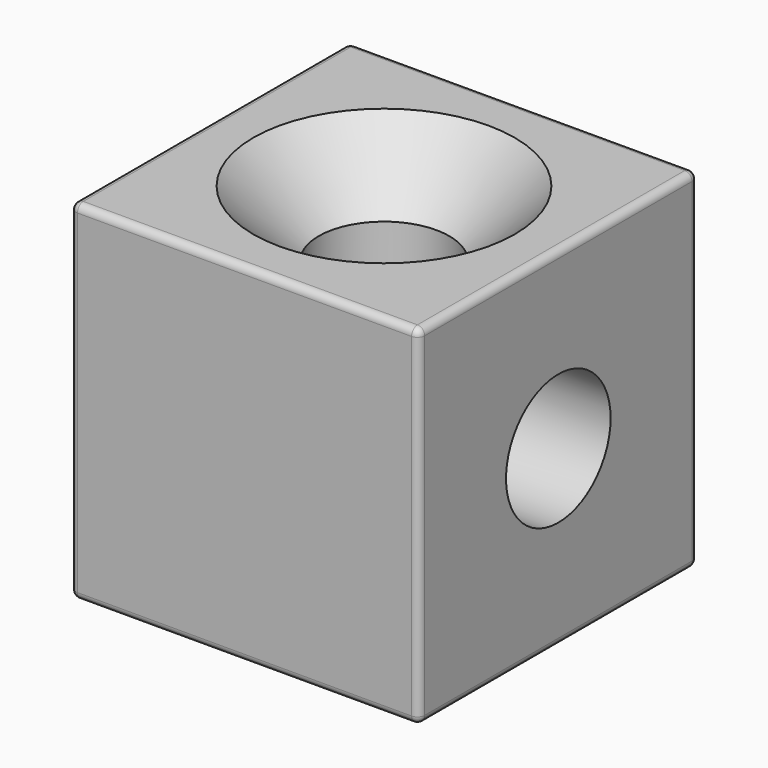
from build123d import *

# Parameters (mm, degrees)
F0_W           = 48
F0_H           = 48
F1_DEPTH       = 48
F2_R           = 1
F3_R           = 1
F4_T1_DEPTH    = 46
F4_T3_DEPTH    = 46
F4_T5_DEPTH    = 46
F4_S9_W        = 1
F4_S9_H        = 1
F4_T10_DEPTH   = 1
F4_S15_W       = 1
F4_S15_H       = 1
F4_T16_DEPTH   = 1
F4_S21_W       = 1
F4_S21_H       = 1
F4_T22_DEPTH   = 1
F4_S27_W       = 1
F4_S27_H       = 1
F4_T28_DEPTH   = 1
F4_T32_ANGLE   = 90
F4_T34_ANGLE   = 90
F6_D           = 18
F6_CSINK_D     = 36
F6_CSINK_ANGLE = 90
F8_D           = 18
F8_CSINK_D     = 36
F8_CSINK_ANGLE = 90


# Not quite as in the source:
# - a fillet or chamfer that OpenCascade refuses, or shapes differently, is made with other operations: its cross-section is extruded or revolved along the edge and cut away or added


with BuildPart() as f1:
    # F0 (on Front) → F1 (new body)
    with BuildSketch(Plane.XZ):
        Rectangle(F0_W, F0_H)
    extrude(amount=F1_DEPTH)

    # F2
    f2_edges = [f1.edges().sort_by_distance(p)[0] for p in [
        (24, -24, 24),
    ]]
    fillet(f2_edges, radius=F2_R)

    # F3
    f3_edges = [f1.edges().sort_by_distance(p)[0] for p in [
        (-24, -24, 24),
        (-0.5, 0, 24),
        (-0.5, -48, 24),
    ]]
    fillet(f3_edges, radius=F3_R)

    # F4: fillet of radius 1 on 8 edges, made by hand

    # F4_s2 → F4_t1 (cut)
    with BuildSketch(Plane.XY.offset(-23)):
        with BuildLine():
            ThreePointArc((-23, -48), (-23.7071067812, -47.7071067812), (-24, -47))
            Line((-24, -47), (-24, -48))
            Line((-24, -48), (-23, -48))
        make_face()
        with BuildLine():
            ThreePointArc((-23, 0), (-23.7071067812, -0.2928932188), (-24, -1))
            Line((-24, -1), (-24, 0))
            Line((-24, 0), (-23, 0))
        make_face()
    extrude(amount=F4_T1_DEPTH, mode=Mode.SUBTRACT)

    # F4_s4 → F4_t3 (cut)
    with BuildSketch(Plane.YZ.offset(-23)):
        with BuildLine():
            ThreePointArc((0, -23), (-0.2928932188, -23.7071067812), (-1, -24))
            Line((-1, -24), (0, -24))
            Line((0, -24), (0, -23))
        make_face()
        with BuildLine():
            ThreePointArc((-48, -23), (-47.7071067812, -23.7071067812), (-47, -24))
            Line((-47, -24), (-48, -24))
            Line((-48, -24), (-48, -23))
        make_face()
    extrude(amount=F4_T3_DEPTH, mode=Mode.SUBTRACT)

    # F4_s6 → F4_t5 (cut)
    with BuildSketch(Plane.XZ.offset(1)):
        with BuildLine():
            ThreePointArc((-24, -23), (-23.7071067812, -23.7071067812), (-23, -24))
            Line((-23, -24), (-24, -24))
            Line((-24, -24), (-24, -23))
        make_face()
        with BuildLine():
            ThreePointArc((24, -23), (23.7071067812, -23.7071067812), (23, -24))
            Line((23, -24), (24, -24))
            Line((24, -24), (24, -23))
        make_face()
    extrude(amount=F4_T5_DEPTH, mode=Mode.SUBTRACT)


with BuildPart() as f4_tool8:
    # F4_s9 → F4_t10 (new body)
    with BuildSketch(Plane.XZ.offset(1)):
        with Locations((-23.5, 23.5)):
            Rectangle(F4_S9_W, F4_S9_H)
    extrude(amount=-F4_T10_DEPTH)

    # F4_s11 → F4_t12 (revolve, cut)
    with BuildSketch(Plane(origin=(-23, -1, 23), x_dir=(0.7071067812, 0, -0.7071067812), z_dir=(0.7071067812, 0, 0.7071067812))):
        with BuildLine():
            ThreePointArc((0, -1), (1, 0), (0, 1))
            Line((0, 1), (0, -1))
        make_face()
    revolve(axis=Axis((-23, -1, 23), (0, 1, 0)), mode=Mode.SUBTRACT)


with BuildPart() as f1_1:
    add(f1.part)

    # F4_t7: cut F4_tool8
    add(f4_tool8.part, mode=Mode.SUBTRACT)


with BuildPart() as f4_tool14:
    # F4_s15 → F4_t16 (new body)
    with BuildSketch(Plane.XZ.offset(47)):
        with Locations((-23.5, 23.5)):
            Rectangle(F4_S15_W, F4_S15_H)
    extrude(amount=F4_T16_DEPTH)

    # F4_s17 → F4_t18 (revolve, cut)
    with BuildSketch(Plane(origin=(-23, -47, 23), x_dir=(0.7071067812, 0, -0.7071067812), z_dir=(-0.7071067812, 0, -0.7071067812))):
        with BuildLine():
            ThreePointArc((0, -1), (1, 0), (0, 1))
            Line((0, 1), (0, -1))
        make_face()
    revolve(axis=Axis((-23, -47, 23), (0, -1, 0)), mode=Mode.SUBTRACT)


with BuildPart() as f1_2:
    add(f1_1.part)

    # F4_t13: cut F4_tool14
    add(f4_tool14.part, mode=Mode.SUBTRACT)


with BuildPart() as f4_tool20:
    # F4_s21 → F4_t22 (new body)
    with BuildSketch(Plane.XZ.offset(47)):
        with Locations((-23.5, -23.5)):
            Rectangle(F4_S21_W, F4_S21_H)
    extrude(amount=F4_T22_DEPTH)

    # F4_s23 → F4_t24 (revolve, cut)
    with BuildSketch(Plane(origin=(-23, -47, -23), x_dir=(0.7071067812, 0, 0.7071067812), z_dir=(0.7071067812, 0, -0.7071067812))):
        with BuildLine():
            ThreePointArc((0, -1), (1, 0), (0, 1))
            Line((0, 1), (0, -1))
        make_face()
    revolve(axis=Axis((-23, -47, -23), (0, -1, 0)), mode=Mode.SUBTRACT)


with BuildPart() as f1_3:
    add(f1_2.part)

    # F4_t19: cut F4_tool20
    add(f4_tool20.part, mode=Mode.SUBTRACT)


with BuildPart() as f4_tool26:
    # F4_s27 → F4_t28 (new body)
    with BuildSketch(Plane.XZ.offset(1)):
        with Locations((-23.5, -23.5)):
            Rectangle(F4_S27_W, F4_S27_H)
    extrude(amount=-F4_T28_DEPTH)

    # F4_s29 → F4_t30 (revolve, cut)
    with BuildSketch(Plane(origin=(-23, -1, -23), x_dir=(0.7071067812, 0, 0.7071067812), z_dir=(-0.7071067812, 0, 0.7071067812))):
        with BuildLine():
            ThreePointArc((0, -1), (1, 0), (0, 1))
            Line((0, 1), (0, -1))
        make_face()
    revolve(axis=Axis((-23, -1, -23), (0, 1, 0)), mode=Mode.SUBTRACT)


with BuildPart() as f1_4:
    add(f1_3.part)

    # F4_t25: cut F4_tool26
    add(f4_tool26.part, mode=Mode.SUBTRACT)

    # F4_s31 → F4_t32 (revolve, cut)
    with BuildSketch(Plane.XZ.offset(1)):
        with BuildLine():
            ThreePointArc((24, -23), (23.7071067812, -23.7071067812), (23, -24))
            Line((23, -24), (24, -24))
            Line((24, -24), (24, -23))
        make_face()
    revolve(axis=Axis((23, -1, -24), (0, 0, 1)), revolution_arc=F4_T32_ANGLE, mode=Mode.SUBTRACT)

    # F4_s33 → F4_t34 (revolve, cut)
    with BuildSketch(Plane.XZ.offset(47)):
        with BuildLine():
            ThreePointArc((24, -23), (23.7071067812, -23.7071067812), (23, -24))
            Line((23, -24), (24, -24))
            Line((24, -24), (24, -23))
        make_face()
    revolve(axis=Axis((23, -47, -24), (0, 0, -1)), revolution_arc=F4_T34_ANGLE, mode=Mode.SUBTRACT)

    # F6 (through all)
    with Locations(Plane.XY.offset(24)):
        with Locations((0, -24)):
            CounterSinkHole(F6_D / 2, F6_CSINK_D / 2, counter_sink_angle=F6_CSINK_ANGLE)

    # F8 (through all)
    with Locations(Plane(origin=(-24, 0, 0), x_dir=(0, -1, 0), z_dir=(-1, 0, 0))):
        with Locations((24, 0)):
            CounterSinkHole(F8_D / 2, F8_CSINK_D / 2, counter_sink_angle=F8_CSINK_ANGLE)


solid = f1_4.part
